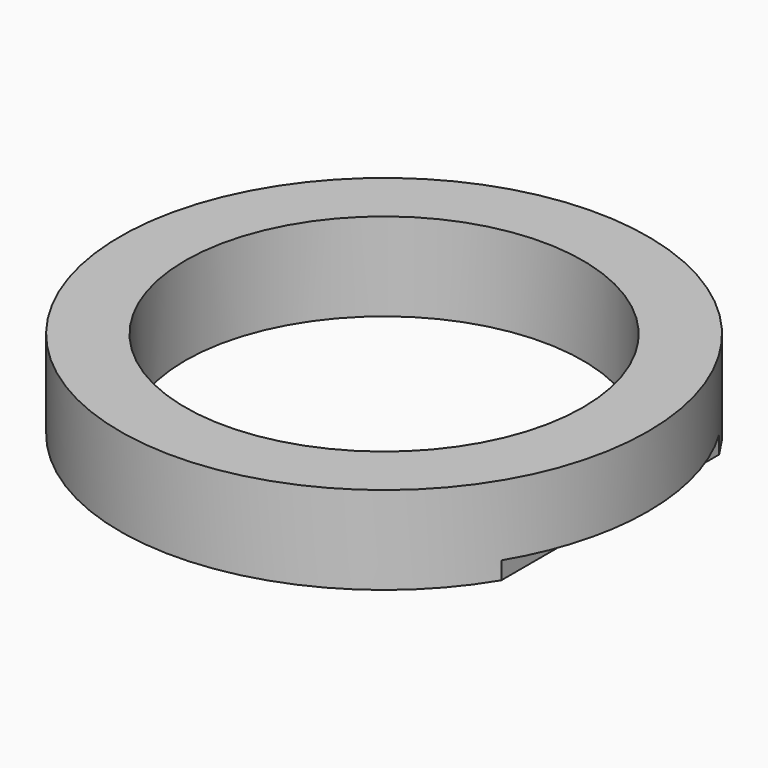
from build123d import *

# Parameters (mm, degrees)
F0_R     = 38.1
F0_R_2   = 28.702
F1_DEPTH = 12.7
F3_DEPTH = 2.54


with BuildPart() as f1:
    # F0 (on Top) → F1 (new body)
    with BuildSketch(Plane.XY):
        Circle(F0_R)
        Circle(F0_R_2, mode=Mode.SUBTRACT)
    extrude(amount=F1_DEPTH)

    # F2 (on face) → F3 (cut)
    with BuildSketch(Plane(origin=(0, 0, 0), x_dir=(1, 0, 0), z_dir=(0, 0, -1))):
        with BuildLine():
            ThreePointArc((38.1, 0), (36.7092304415, 10.2001176655), (32.6384566724, 19.6555627251))
            Line((32.6384566724, 19.6555627251), (32.6384566724, -19.6555627251))
            ThreePointArc((32.6384566724, -19.6555627251), (36.7092304415, -10.2001176655), (38.1, 0))
        make_face()
        with BuildLine():
            Line((45.6830970943, -36.9560495019), (45.6830970943, 39.5725145936))
            Line((45.6830970943, 39.5725145936), (32.6384566724, 39.5725145936))
            Line((32.6384566724, 39.5725145936), (32.6384566724, 19.6555627251))
            ThreePointArc((32.6384566724, 19.6555627251), (36.7092304415, 10.2001176655), (38.1, 0))
            ThreePointArc((38.1, 0), (36.7092304415, -10.2001176655), (32.6384566724, -19.6555627251))
            Line((32.6384566724, -19.6555627251), (32.6384566724, -36.9560495019))
            Line((32.6384566724, -36.9560495019), (45.6830970943, -36.9560495019))
        make_face()
    extrude(amount=-F3_DEPTH, mode=Mode.SUBTRACT)


solid = f1.part
